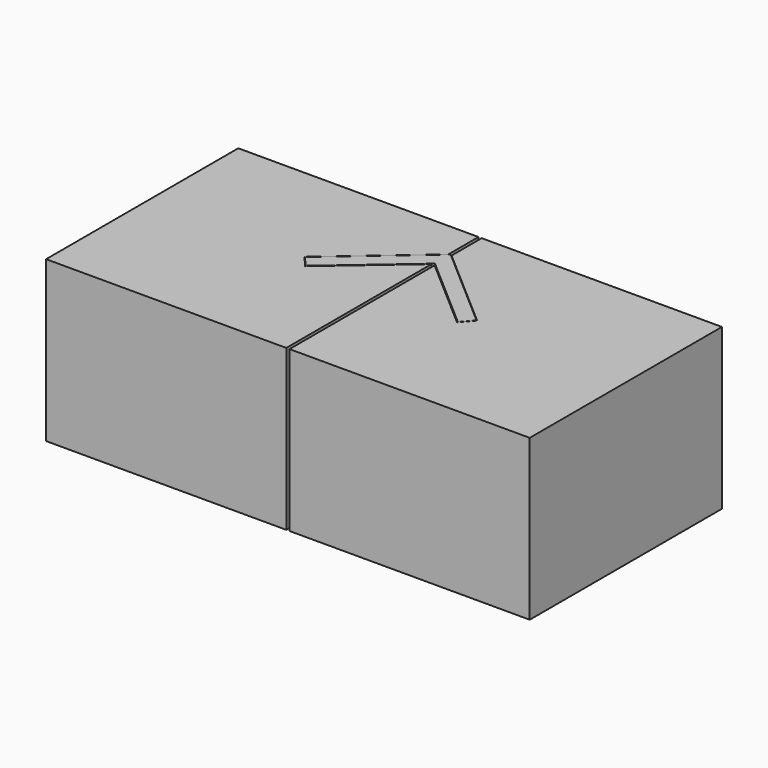
from build123d import *

# Parameters (mm, degrees)
F1_DEPTH = 20
F3_DEPTH = 20


# Not quite as in the source:
# - ends of sketch curves that miss each other by under 0.0002 mm in the source are joined


with BuildPart() as f1:
    # F0 (on Top) → F1 (new body)
    with BuildSketch(Plane.XY):
        Polygon((-0.2, 19.9680037051), (-30.2, 19.9680037051), (-30.2, -10.0319962949), (-0.2, -10.0319962949), (-0.2, 12.6258979241), (-9.537948603, 4.5824087189), (-10.8432257548, 6.0977474786), (-0.2, 15.2655717093), align=None)
    extrude(amount=F1_DEPTH)


with BuildPart() as f1b:
    # F0 (on Top) → F1, piece 2 (new body)
    with BuildSketch(Plane.XY):
        Polygon((0.2, 19.9680037051), (0.2, 15.2637217937), (10.7280267403, 6.0977474786), (9.4147583618, 4.5893290465), (0.2, 12.6119377033), (0.2, -10.0319962949), (30.2, -10.0319962949), (30.2, 19.9680037051), align=None)
    extrude(amount=F1_DEPTH)


with BuildPart() as f3:
    # F2 (on Top) → F3 (new body)
    with BuildSketch(Plane.XY):
        Polygon((-10.772710357, 6.0924959384), (-9.5653289916, 4.6908075856), (-0.0066424788, 12.9244352324), (9.44271132, 4.6975816776), (10.65748457, 6.0928687273), (-0.0001748021, 15.3717045883), align=None)
    extrude(amount=F3_DEPTH)


solid = Compound([f1.part, f1b.part, f3.part])
